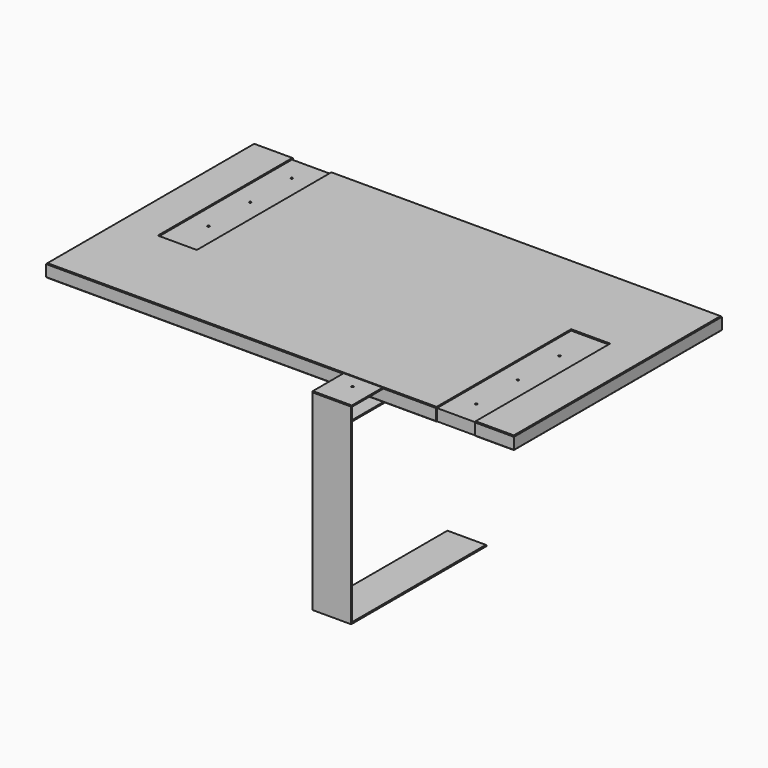
from build123d import *

# Parameters (mm, degrees)
F0_W      = 1800
F0_H      = 1000
F1_DEPTH  = 50
F2_W      = 150
F2_H      = 10
F3_DEPTH  = 650
F4_W      = 150
F4_H      = 5
F5_DEPTH  = 650
F6_R      = 4
F7_DEPTH  = 50
F8_W      = 150
F8_H      = 5
F9_DEPTH  = 650
F10_W     = 150
F10_H     = 5
F11_DEPTH = 735
F12_W     = 150
F12_H     = 5
F13_DEPTH = 645
F14_W     = 150
F14_H     = 5
F15_DEPTH = 645
F16_R     = 4
F17_DEPTH = 80
F18_W     = 150
F18_H     = 5
F19_DEPTH = 100
F20_W     = 150
F20_H     = 5
F21_DEPTH = 100
F22_SIZE  = 3
F23_SIZE  = 3
F24_SIZE  = 1


with BuildPart() as f1:
    # F0 (on Top) → F1 (new body)
    with BuildSketch(Plane.XY):
        Rectangle(F0_W, F0_H)
    extrude(amount=F1_DEPTH)

    # F2 (on face) → F3 (cut)
    with BuildSketch(Plane.XZ.offset(500)):
        with Locations((675, 50)):
            Rectangle(F2_W, F2_H)
    extrude(amount=-F3_DEPTH, mode=Mode.SUBTRACT)

    # F4 (on face) → F5 (cut)
    with BuildSketch(Plane(origin=(0, 500, 0), x_dir=(-1, 0, 0), z_dir=(0, 1, 0))):
        with Locations((675, 47.5)):
            Rectangle(F4_W, F4_H)
    extrude(amount=-F5_DEPTH, mode=Mode.SUBTRACT)

    # F6 (on face) → F7 (cut)
    with BuildSketch(Plane.XY.offset(45)):
        with Locations((675, 0)):
            Circle(F6_R)
        with Locations((675, -200)):
            Circle(F6_R)
        with Locations((675, -400)):
            Circle(F6_R)
        with Locations((-675, 400)):
            Circle(F6_R)
        with Locations((-675, 200)):
            Circle(F6_R)
        with Locations((-675, 0)):
            Circle(F6_R)
    extrude(amount=-F7_DEPTH, mode=Mode.SUBTRACT)

    # F18 (on face) → F19 (cut)
    with BuildSketch(Plane.XY.offset(45)):
        with Locations((675, -497.5)):
            Rectangle(F18_W, F18_H)
    extrude(amount=-F19_DEPTH, mode=Mode.SUBTRACT)

    # F20 (on face) → F21 (cut)
    with BuildSketch(Plane.XY.offset(45)):
        with Locations((-675, 497.5)):
            Rectangle(F20_W, F20_H)
    extrude(amount=-F21_DEPTH, mode=Mode.SUBTRACT)

    # F22
    f22_edges = [f1.edges().sort_by_distance(p)[0] for p in [
        (150, 500, 50),
        (-825, 500, 50),
        (-900, 0, 50),
        (-150, -500, 50),
        (825, -500, 50),
        (825, -500, 0),
        (-150, -500, 0),
        (-900, 0, 0),
        (-825, 500, 0),
        (150, 500, 0),
        (900, 0, 50),
        (900, 0, 0),
    ]]
    chamfer(f22_edges, length=F22_SIZE)


with BuildPart() as f9:
    # F8 (on Front) → F9 (new body)
    with BuildSketch(Plane.XZ):
        with Locations((318.7353536487, 46.0768144429)):
            Rectangle(F8_W, F8_H)
    extrude(amount=F9_DEPTH)

    # F10 (on face) → F11 (join)
    with BuildSketch(Plane(origin=(0, 0, 43.5768144429), x_dir=(1, 0, 0), z_dir=(0, 0, -1))):
        with Locations((318.7353536487, 647.5)):
            Rectangle(F10_W, F10_H)
    extrude(amount=F11_DEPTH)

    # F12 (on face) → F13 (join)
    with BuildSketch(Plane(origin=(0, -645, 0), x_dir=(-1, 0, 0), z_dir=(0, 1, 0))):
        with Locations((-318.7353536487, -688.9231855571)):
            Rectangle(F12_W, F12_H)
    extrude(amount=F13_DEPTH)

    # F14 (on face) → F15 (join)
    with BuildSketch(Plane(origin=(0, -645, 0), x_dir=(-1, 0, 0), z_dir=(0, 1, 0))):
        with Locations((-318.7353536487, -3.9231855571)):
            Rectangle(F14_W, F14_H)
    extrude(amount=F15_DEPTH)

    # F16 (on face) → F17 (cut)
    with BuildSketch(Plane.XY.offset(48.5768144429)):
        with Locations((318.7353536487, -150)):
            Circle(F16_R)
        with Locations((318.7353536487, -350)):
            Circle(F16_R)
        with Locations((318.7353536487, -550)):
            Circle(F16_R)
    extrude(amount=-F17_DEPTH, mode=Mode.SUBTRACT)

    # F23
    f23_edges = [f9.edges().sort_by_distance(p)[0] for p in [
        (318.735354, -650, 48.576814),
    ]]
    chamfer(f23_edges, length=F23_SIZE)

    # F24
    f24_edges = [f9.edges().sort_by_distance(p)[0] for p in [
        (393.735354, -650, -322.923186),
        (243.735354, -650, -322.923186),
        (243.735354, -645, -346.423186),
        (393.735354, -645, -346.423186),
        (318.735354, 0, -686.423186),
        (393.735354, -322.5, -686.423186),
        (243.735354, -322.5, -686.423186),
    ]]
    chamfer(f24_edges, length=F24_SIZE)


solid = Compound([f1.part, f9.part])
